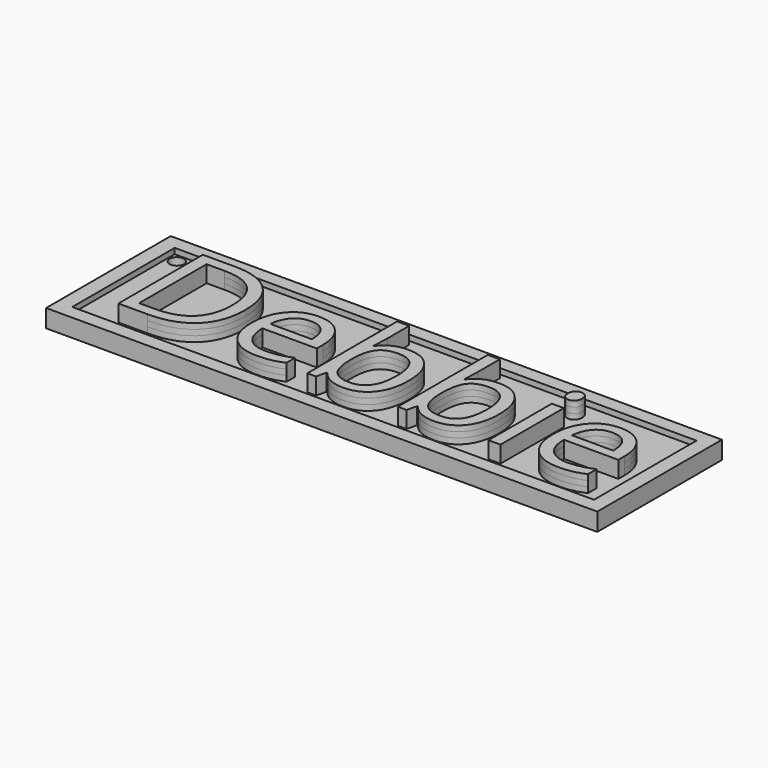
from build123d import *

# Parameters (mm, degrees)
F0_W         = 125.2244971693
F0_H         = 35.3852584958
F1_DEPTH     = 4.064
F2_W         = 118.5406185687
F2_H         = 29.0945451707
F3_DEPTH     = 1.27
F4_TEXT_SIZE = 33.5832307529
F5_DEPTH     = 4.064
F6_R         = 1.6519059461
F7_DEPTH     = 25.4
F8_DEPTH     = 1.27
F9_DEPTH     = 2.54


# Not quite as in the source:
# - Text() gives the source's letters only with a copy of the font that has no kerning and outlines rounded to 1/6400 em; it was checked with that copy


with BuildPart() as f1:
    # F0 (on Top) → F1 (new body)
    with BuildSketch(Plane.XY):
        with Locations((1.3354290277, 1.0289419442)):
            Rectangle(F0_W, F0_H)
    extrude(amount=F1_DEPTH)

    # F2 (on face) → F3 (cut)
    with BuildSketch(Plane.XY.offset(4.064)):
        with Locations((1.3760942966, 1.081216149)):
            Rectangle(F2_W, F2_H)
    extrude(amount=-F3_DEPTH, mode=Mode.SUBTRACT)

    # F4 (on face) → F5 (join)
    with BuildSketch(Plane.XY.offset(4.064)):
        with Locations((-52.5864250958, -11.1070387065)):
            Text('Debbie', F4_TEXT_SIZE, font='Open Sans', text_align=(TextAlign.LEFT, TextAlign.BOTTOM))
    extrude(amount=-F5_DEPTH)

    # F6 (on face) → F7 (cut)
    with BuildSketch(Plane.XY.offset(4.064)):
        with Locations((-55.8572895825, 13.6816818267)):
            Circle(F6_R)
    extrude(amount=-F7_DEPTH, mode=Mode.SUBTRACT)

    # F4 (on face) → F8 (join)
    with BuildSketch(Plane.XY.offset(4.064)):
        with Locations((-52.5864250958, -11.1070387065)):
            Text('Debbie', F4_TEXT_SIZE, font='Open Sans', text_align=(TextAlign.LEFT, TextAlign.BOTTOM))
    extrude(amount=F8_DEPTH)

    # F4 (on face) → F9 (join)
    with BuildSketch(Plane.XY.offset(4.064)):
        with Locations((-52.5864250958, -11.1070387065)):
            Text('Debbie', F4_TEXT_SIZE, font='Open Sans', text_align=(TextAlign.LEFT, TextAlign.BOTTOM))
    extrude(amount=F9_DEPTH)


solid = f1.part
